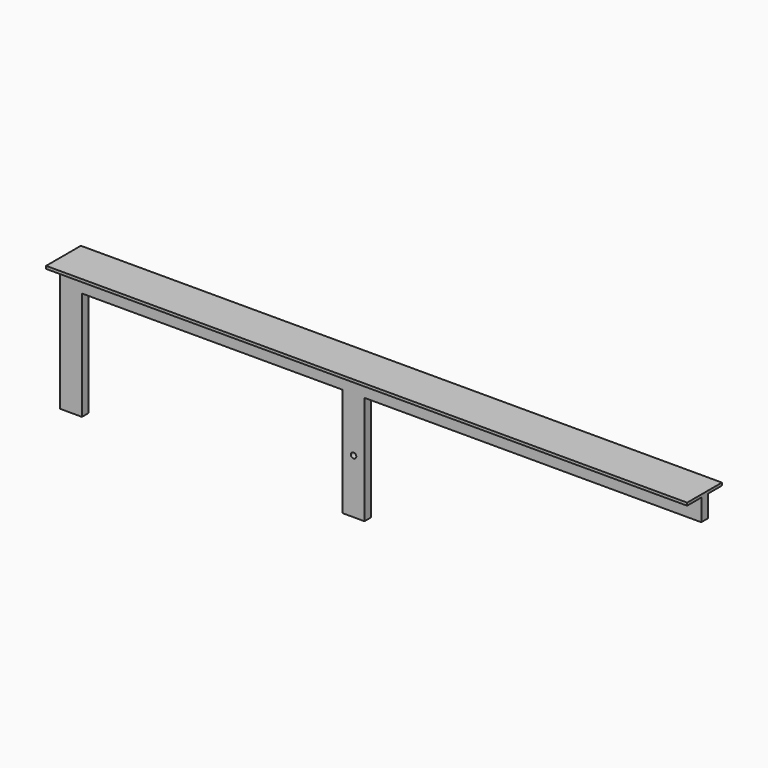
from build123d import *

# Parameters (mm, degrees)
F0_W     = 393.7
F0_H     = 25.4
F0_W_2   = 25.4
F0_H_2   = 127
F0_W_3   = 304.8
F1_DEPTH = 9.525
F2_W     = 749.3
F2_H     = 20.6375
F2_H_2   = 9.525
F3_DEPTH = 3.175
F4_R     = 3.175
F5_DEPTH = 30.1635


with BuildPart() as f1:
    # F0 (on Front) → F1 (new body)
    with BuildSketch(Plane.XZ):
        with Locations((-132.7033620834, -20.5259278297)):
            Rectangle(F0_W, F0_H)
        with Locations((-342.2533620834, -20.5259278297)):
            Rectangle(F0_W_2, F0_H)
        with Locations((-342.2533620834, -96.7259278297)):
            Rectangle(F0_W_2, F0_H_2)
        with Locations((-507.3533620834, -20.5259278297)):
            Rectangle(F0_W_3, F0_H)
        with Locations((-672.4533620834, -20.5259278297)):
            Rectangle(F0_W_2, F0_H)
        with Locations((-672.4533620834, -96.7259278297)):
            Rectangle(F0_W_2, F0_H_2)
    extrude(amount=F1_DEPTH)

    # F2 (on face) → F3 (join)
    with BuildSketch(Plane.XY.offset(-7.8259278297)):
        with Locations((-310.5033620834, 10.31875)):
            Rectangle(F2_W, F2_H)
        with Locations((-310.5033620834, -4.7625)):
            Rectangle(F2_W, F2_H_2)
        with Locations((-310.5033620834, -19.84375)):
            Rectangle(F2_W, F2_H)
    extrude(amount=F3_DEPTH)

    # F4 (on face) → F5 (cut, through all)
    with BuildSketch(Plane.XZ.offset(9.525)):
        with Locations((-342.2533620834, -96.7259278297)):
            Circle(F4_R)
    extrude(amount=-F5_DEPTH, mode=Mode.SUBTRACT)


solid = f1.part
